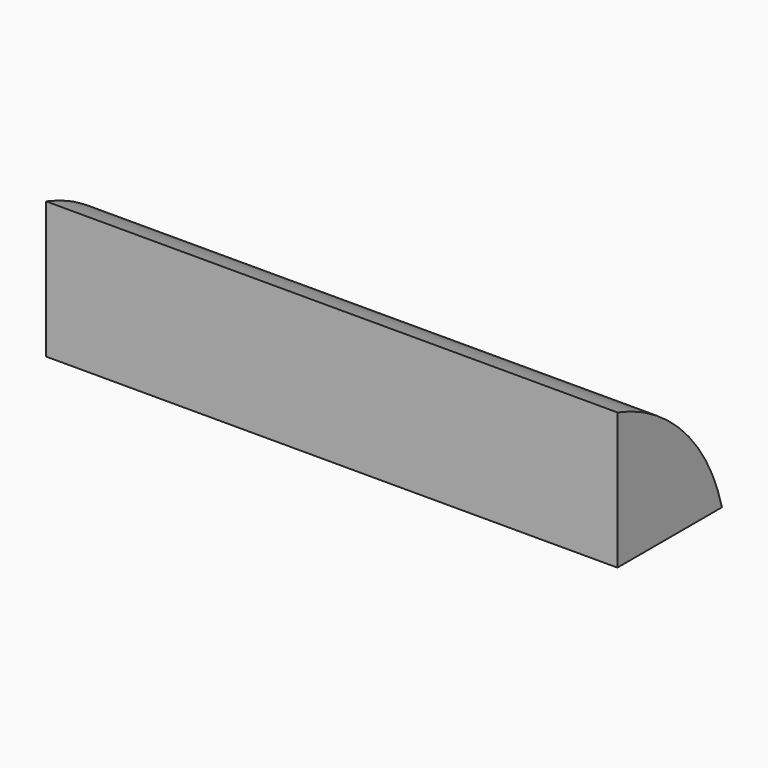
from build123d import *

# Parameters (mm, degrees)
F0_W        = 7.112
F0_H        = 1.8034
F1_DEPTH    = 1.6256
F2_T1_DEPTH = 18.7023867637
F3_W        = 6.6736862063
F3_H        = 0.8746144013
F4_DEPTH    = 0.5334


# Not quite as in the source:
# - a fillet or chamfer that OpenCascade refuses, or shapes differently, is made with other operations: its cross-section is extruded or revolved along the edge and cut away or added


with BuildPart() as f1:
    # F0 (on Front) → F1 (new body)
    with BuildSketch(Plane.XZ):
        with Locations((-59.9939581946, 49.5912485233)):
            Rectangle(F0_W, F0_H)
    extrude(amount=-F1_DEPTH)

    # F2: fillet of radius 2.3915199549 on 1 edges, made by hand

    # F2_s2 → F2_t1 (cut)
    with BuildSketch(Plane.YZ.offset(-69.3451515765)):
        with BuildLine():
            ThreePointArc((-0.6924773527, 50.4929485233), (0.7760026585, 49.9890021832), (1.6256, 48.6895485233))
            Line((1.6256, 48.6895485233), (1.6719615471, 48.7013109224))
            ThreePointArc((1.6719615471, 48.7013109224), (1.6734303991, 49.5912485233), (1.6734303991, 50.4929485233))
            Line((1.6734303991, 50.4929485233), (1.6256, 50.5407789224))
            Line((1.6256, 50.5407789224), (-0.6924773527, 50.5407789224))
            Line((-0.6924773527, 50.5407789224), (-0.6924773527, 50.4929485233))
        make_face()
    extrude(amount=F2_T1_DEPTH, mode=Mode.SUBTRACT)

    # F3 (on face) → F4 (cut)
    with BuildSketch(Plane(origin=(0, 0, 48.6895485233), x_dir=(1, 0, 0), z_dir=(0, 0, -1))):
        with Locations((-60.0108616054, -0.7537669444)):
            Rectangle(F3_W, F3_H)
    extrude(amount=-F4_DEPTH, mode=Mode.SUBTRACT)


solid = f1.part
